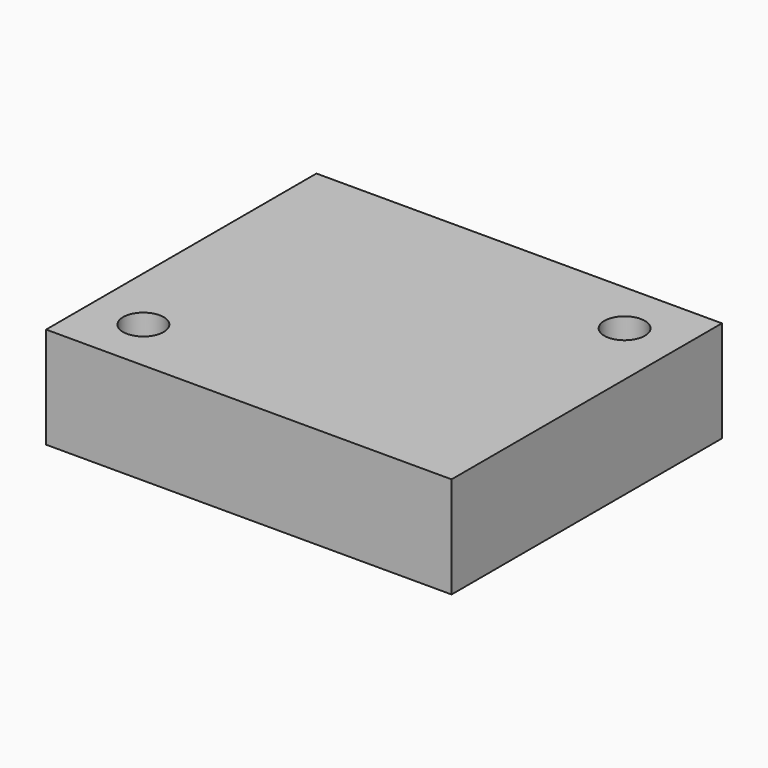
from build123d import *

# Parameters (mm, degrees)
F0_W     = 60
F0_H     = 50
F1_DEPTH = 15
F3_D     = 6
F3_DEPTH = 12
F3_TIP   = 1.8025818571


with BuildPart() as f1:
    # F0 (on Top) → F1 (new body)
    with BuildSketch(Plane.XY):
        Rectangle(F0_W, F0_H)
    extrude(amount=F1_DEPTH)

    # F3
    with Locations(Plane.XY.offset(15)):
        with Locations((-22, -17), (22, 17)):
            Hole(F3_D / 2, depth=F3_DEPTH)
            with Locations((0, 0, -(F3_DEPTH + F3_TIP / 2))):  # 118° drill point
                Cone(0, F3_D / 2, F3_TIP, mode=Mode.SUBTRACT)


solid = f1.part
